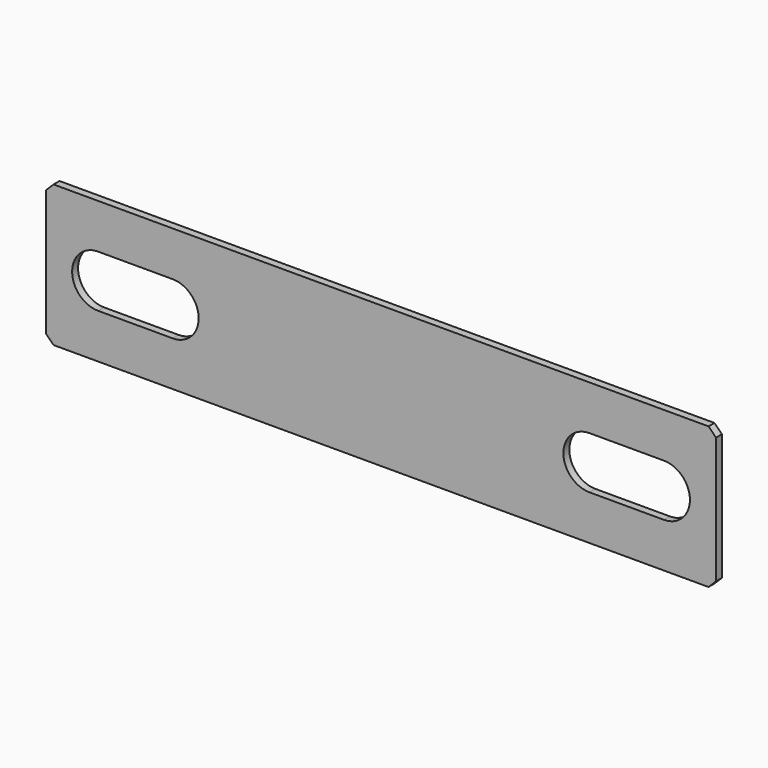
from build123d import *

# Parameters (mm, degrees)
F0_W     = 90
F0_H     = 19
F1_DEPTH = 1
F2_SIZE  = 1
F3_SIZE  = 1
F4_SIZE  = 1
F5_SIZE  = 1


# Not quite as in the source:
# - ends of sketch curves that miss each other by under 0.0002 mm in the source are joined


with BuildPart() as f1:
    # F0 (on Front) → F1 (new body)
    with BuildSketch(Plane.XZ):
        with Locations((45, 9.5)):
            Rectangle(F0_W, F0_H)
        with BuildLine():
            Line((17, 6), (7, 6))
            ThreePointArc((7, 6), (3.5, 9.5), (7, 13))
            Line((7, 13), (17, 13))
            ThreePointArc((17, 13), (20.4999967813, 9.5), (17, 6))
        make_face(mode=Mode.SUBTRACT)
        with BuildLine():
            ThreePointArc((83, 13), (86.5, 9.5), (83, 6))
            Line((83, 6), (73.0000032187, 6))
            ThreePointArc((73.0000032187, 6), (69.5000032187, 9.5), (73.0000032187, 13))
            Line((73.0000032187, 13), (83, 13))
        make_face(mode=Mode.SUBTRACT)
    extrude(amount=F1_DEPTH)

    # F2
    f2_edges = [f1.edges().sort_by_distance(p)[0] for p in [
        (90, -0.5, 19),
    ]]
    chamfer(f2_edges, length=F2_SIZE)

    # F3
    f3_edges = [f1.edges().sort_by_distance(p)[0] for p in [
        (90, -0.5, 0),
    ]]
    chamfer(f3_edges, length=F3_SIZE)

    # F4
    f4_edges = [f1.edges().sort_by_distance(p)[0] for p in [
        (0, -0.5, 19),
    ]]
    chamfer(f4_edges, length=F4_SIZE)

    # F5
    f5_edges = [f1.edges().sort_by_distance(p)[0] for p in [
        (0, -0.5, 0),
    ]]
    chamfer(f5_edges, length=F5_SIZE)


solid = f1.part
